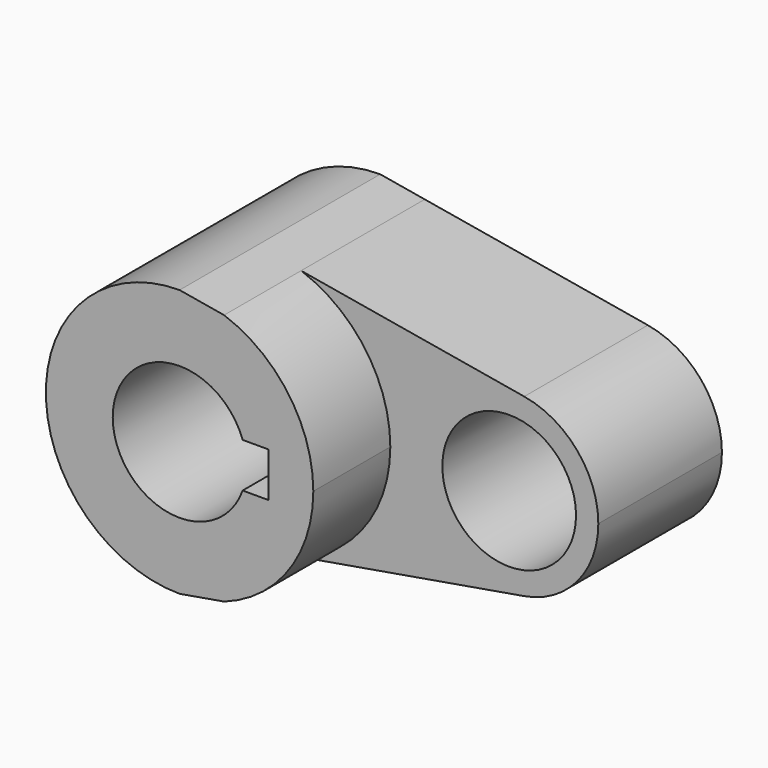
from build123d import *

# Parameters (mm, degrees)
F0_R     = 14.2875
F1_DEPTH = 33.02
F2_DEPTH = 53.594


with BuildPart() as f1:
    # F0 (on Front) → F1 (new body)
    with BuildSketch(Plane.XZ):
        with BuildLine():
            Line((9.5121844836, 26.9452959039), (0, 28.575))
            ThreePointArc((0, 28.575), (-28.575, 0), (0, -28.575))
            Line((0, -28.575), (9.5121844836, -26.9452959039))
            ThreePointArc((9.5121844836, -26.9452959039), (23.3274655355, -16.5033322905), (28.575, 0))
            ThreePointArc((28.575, 0), (23.3274655355, 16.5033322905), (9.5121844836, 26.9452959039))
        make_face()
        with BuildLine():
            ThreePointArc((-13.4703841816, 4.7625), (0, 14.2875), (13.4703841816, 4.7625))
            Line((13.4703841816, 4.7625), (19.05, 4.7625))
            Line((19.05, 4.7625), (19.05, -4.7625))
            Line((19.05, -4.7625), (13.4703841816, -4.7625))
            ThreePointArc((13.4703841816, -4.7625), (0, -14.2875), (-13.4703841816, -4.7625))
            Line((-13.4703841816, -4.7625), (-19.05, -4.7625))
            Line((-19.05, -4.7625), (-19.05, 4.7625))
            Line((-19.05, 4.7625), (-13.4703841816, 4.7625))
        make_face(mode=Mode.SUBTRACT)
        with BuildLine():
            Line((57.1919272622, 18.7764181619), (9.5121844836, 26.9452959039))
            ThreePointArc((9.5121844836, 26.9452959039), (23.3274655355, 16.5033322905), (28.575, 0))
            ThreePointArc((28.575, 0), (23.3274655355, -16.5033322905), (9.5121844836, -26.9452959039))
            Line((9.5121844836, -26.9452959039), (57.1919272622, -18.7764181619))
            ThreePointArc((57.1919272622, -18.7764181619), (34.925, 0), (57.1919272622, 18.7764181619))
        make_face()
        with BuildLine():
            ThreePointArc((73.025, 0), (68.5383952831, 12.2804730295), (57.1919272622, 18.7764181619))
            ThreePointArc((57.1919272622, 18.7764181619), (34.925, 0), (57.1919272622, -18.7764181619))
            ThreePointArc((57.1919272622, -18.7764181619), (68.5383952831, -12.2804730295), (73.025, 0))
        make_face()
        with Locations((53.975, 0)):
            Circle(F0_R, mode=Mode.SUBTRACT)
        with BuildLine():
            ThreePointArc((-13.4703841816, -4.7625), (-14.2875, 0), (-13.4703841816, 4.7625))
            Line((-13.4703841816, 4.7625), (-19.05, 4.7625))
            Line((-19.05, 4.7625), (-19.05, -4.7625))
            Line((-19.05, -4.7625), (-13.4703841816, -4.7625))
        make_face()
    extrude(amount=F1_DEPTH)

    # F0 (on Front) → F2 (join)
    with BuildSketch(Plane.XZ):
        with BuildLine():
            Line((9.5121844836, 26.9452959039), (0, 28.575))
            ThreePointArc((0, 28.575), (-28.575, 0), (0, -28.575))
            Line((0, -28.575), (9.5121844836, -26.9452959039))
            ThreePointArc((9.5121844836, -26.9452959039), (23.3274655355, -16.5033322905), (28.575, 0))
            ThreePointArc((28.575, 0), (23.3274655355, 16.5033322905), (9.5121844836, 26.9452959039))
        make_face()
        with BuildLine():
            ThreePointArc((-13.4703841816, 4.7625), (0, 14.2875), (13.4703841816, 4.7625))
            Line((13.4703841816, 4.7625), (19.05, 4.7625))
            Line((19.05, 4.7625), (19.05, -4.7625))
            Line((19.05, -4.7625), (13.4703841816, -4.7625))
            ThreePointArc((13.4703841816, -4.7625), (0, -14.2875), (-13.4703841816, -4.7625))
            Line((-13.4703841816, -4.7625), (-19.05, -4.7625))
            Line((-19.05, -4.7625), (-19.05, 4.7625))
            Line((-19.05, 4.7625), (-13.4703841816, 4.7625))
        make_face(mode=Mode.SUBTRACT)
        with BuildLine():
            ThreePointArc((-13.4703841816, -4.7625), (-14.2875, 0), (-13.4703841816, 4.7625))
            Line((-13.4703841816, 4.7625), (-19.05, 4.7625))
            Line((-19.05, 4.7625), (-19.05, -4.7625))
            Line((-19.05, -4.7625), (-13.4703841816, -4.7625))
        make_face()
    extrude(amount=F2_DEPTH)


solid = f1.part
